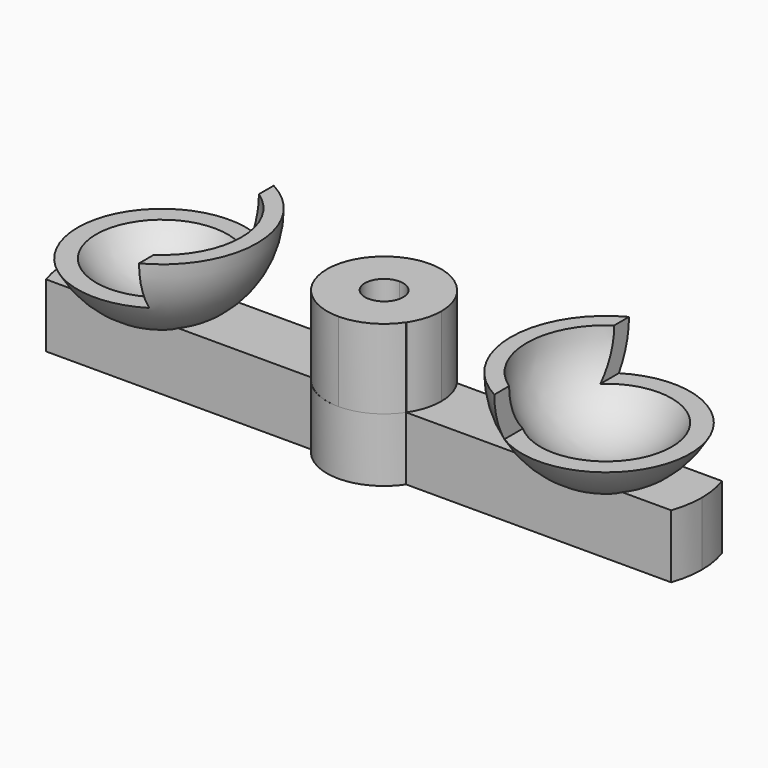
from build123d import *

# Parameters (mm, degrees)
F1_R     = 3
F2_DEPTH = 10
F6_W     = 34.5020639661
F6_H     = 49.154933542
F7_DEPTH = 7
F9_DEPTH = 12.5


with BuildPart() as f2:
    # F1 (on Top) → F2 (new body)
    with BuildSketch(Plane.XY):
        with BuildLine():
            ThreePointArc((46.4564392374, 5), (47.2363289116, 2.5538705461), (47.5, 0))
            ThreePointArc((47.5, 0), (47.2363289116, -2.5538705461), (46.4564392374, -5))
            Line((46.4564392374, -5), (49.2615084811, -5))
            ThreePointArc((49.2615084811, -5), (49.8983064719, -2.5359590739), (50.1125981935, 0))
            ThreePointArc((50.1125981935, 0), (49.8983064719, 2.5359590739), (49.2615084811, 5))
            Line((49.2615084811, 5), (46.4564392374, 5))
        make_face()
        with BuildLine():
            Line((-46.4564392374, 5), (-49.2629836635, 5))
            ThreePointArc((-49.2629836635, 5), (-50.1139903065, 0), (-49.2629836635, -5))
            Line((-49.2629836635, -5), (-46.4564392374, -5))
            ThreePointArc((-46.4564392374, -5), (-47.5, 0), (-46.4564392374, 5))
        make_face()
        with BuildLine():
            ThreePointArc((-22.5, 0), (-22.7636710884, 2.5538705461), (-23.5435607626, 5))
            Line((-23.5435607626, 5), (-46.4564392374, 5))
            ThreePointArc((-46.4564392374, 5), (-47.5, 0), (-46.4564392374, -5))
            Line((-46.4564392374, -5), (-23.5435607626, -5))
            ThreePointArc((-23.5435607626, -5), (-22.7636710884, -2.5538705461), (-22.5, 0))
        make_face()
        with BuildLine():
            ThreePointArc((-19.8860096935, 0), (-20.1002802071, 2.5359521046), (-20.7370163365, 5))
            Line((-20.7370163365, 5), (-23.5435607626, 5))
            ThreePointArc((-23.5435607626, 5), (-22.7636710884, 2.5538705461), (-22.5, 0))
            ThreePointArc((-22.5, 0), (-22.7636710884, -2.5538705461), (-23.5435607626, -5))
            Line((-23.5435607626, -5), (-20.7370163365, -5))
            ThreePointArc((-20.7370163365, -5), (-20.1002802071, -2.5359521046), (-19.8860096935, 0))
        make_face()
        with BuildLine():
            ThreePointArc((-7.4833147735, -5), (-9, 0), (-7.4833147735, 5))
            Line((-7.4833147735, 5), (-20.7370163365, 5))
            ThreePointArc((-20.7370163365, 5), (-20.1002802071, 2.5359521046), (-19.8860096935, 0))
            ThreePointArc((-19.8860096935, 0), (-20.1002802071, -2.5359521046), (-20.7370163365, -5))
            Line((-20.7370163365, -5), (-7.4833147735, -5))
        make_face()
        with BuildLine():
            ThreePointArc((9, 0), (8.6124860802, 2.6124860802), (7.4833147735, 5))
            Line((7.4833147735, 5), (-7.4833147735, 5))
            ThreePointArc((-7.4833147735, 5), (-9, 0), (-7.4833147735, -5))
            Line((-7.4833147735, -5), (7.4833147735, -5))
            ThreePointArc((7.4833147735, -5), (8.6124860802, -2.6124860802), (9, 0))
        make_face()
        Circle(F1_R, mode=Mode.SUBTRACT)
        with BuildLine():
            ThreePointArc((20.7384915189, -5), (19.8874018065, 0), (20.7384915189, 5))
            Line((20.7384915189, 5), (7.4833147735, 5))
            ThreePointArc((7.4833147735, 5), (8.6124860802, 2.6124860802), (9, 0))
            ThreePointArc((9, 0), (8.6124860802, -2.6124860802), (7.4833147735, -5))
            Line((7.4833147735, -5), (20.7384915189, -5))
        make_face()
        with BuildLine():
            ThreePointArc((23.5435607626, -5), (22.5, 0), (23.5435607626, 5))
            Line((23.5435607626, 5), (20.7384915189, 5))
            ThreePointArc((20.7384915189, 5), (19.8874018065, 0), (20.7384915189, -5))
            Line((20.7384915189, -5), (23.5435607626, -5))
        make_face()
        with BuildLine():
            ThreePointArc((46.4564392374, -5), (47.2363289116, -2.5538705461), (47.5, 0))
            ThreePointArc((47.5, 0), (47.2363289116, 2.5538705461), (46.4564392374, 5))
            Line((46.4564392374, 5), (23.5435607626, 5))
            ThreePointArc((23.5435607626, 5), (22.5, 0), (23.5435607626, -5))
            Line((23.5435607626, -5), (46.4564392374, -5))
        make_face()
        with BuildLine():
            Line((-7.4833147735, 5), (7.4833147735, 5))
            ThreePointArc((7.4833147735, 5), (0, 9), (-7.4833147735, 5))
        make_face()
        with BuildLine():
            ThreePointArc((-7.4833147735, -5), (0, -9), (7.4833147735, -5))
            Line((7.4833147735, -5), (-7.4833147735, -5))
        make_face()
    extrude(amount=F2_DEPTH)

    # F8 (on face) → F9 (join)
    with BuildSketch(Plane.XY.offset(10)):
        with BuildLine():
            ThreePointArc((9.0266954303, 0), (8.6391815104, 2.6124860802), (7.5100102038, 5))
            Line((7.5100102038, 5), (7.4833147735, 5))
            ThreePointArc((7.4833147735, 5), (4.2485253114, 7.9341056634), (0.0133477151, 8.9999901021))
            ThreePointArc((0.0133477151, 8.9999901021), (-8.9733045697, 0), (0.0133477151, -8.9999901021))
            ThreePointArc((0.0133477151, -8.9999901021), (4.2485253114, -7.9341056634), (7.4833147735, -5))
            Line((7.4833147735, -5), (7.5100102038, -5))
            ThreePointArc((7.5100102038, -5), (8.6391815104, -2.6124860802), (9.0266954303, 0))
        make_face()
        with BuildLine():
            ThreePointArc((0.0133477151, 2.9999703063), (2.1432913831, 2.126034236), (3.0266954303, 0))
            ThreePointArc((3.0266954303, 0), (2.1432913831, -2.126034236), (0.0133477151, -2.9999703063))
            ThreePointArc((0.0133477151, -2.9999703063), (-3, 0), (0.0133477151, 2.9999703063))
        make_face(mode=Mode.SUBTRACT)
    extrude(amount=F9_DEPTH)


with BuildPart() as f4:
    # F3 (on Front) → F4 (revolve)
    with BuildSketch(Plane.XZ):
        with BuildLine():
            Line((-47.5, 22.5), (-50, 22.5))
            ThreePointArc((-50, 22.5), (-45.6066017178, 11.8933982822), (-35, 7.5))
            Line((-35, 7.5), (-35, 10))
            ThreePointArc((-35, 10), (-43.8388347648, 13.6611652352), (-47.5, 22.5))
        make_face()
    revolve(axis=Axis((-35, 0, 15.5329470341), (0, 0, 1)))


with BuildPart() as f5:
    # F3 (on Front) → F5 (revolve)
    with BuildSketch(Plane.XZ):
        with BuildLine():
            Line((22.5, 22.5), (20, 22.5))
            ThreePointArc((20, 22.5), (24.3933982822, 11.8933982822), (35, 7.5))
            Line((35, 7.5), (35, 10))
            ThreePointArc((35, 10), (26.1611652352, 13.6611652352), (22.5, 22.5))
        make_face()
    revolve(axis=Axis((35, 0, 11.25), (0, 0, -1)))


with BuildPart() as f7_tool:
    # F6 (on face) → F7 (new body)
    with BuildSketch(Plane.XY.offset(22.5)):
        with BuildLine():
            Line((28, 25.6732665002), (28, 13.2664991614))
            ThreePointArc((28, 13.2664991614), (42.7459666924, 12.8452325787), (50, 0))
            ThreePointArc((50, 0), (42.7459666924, -12.8452325787), (28, -13.2664991614))
            Line((28, -13.2664991614), (28, -23.4816670418))
            Line((28, -23.4816670418), (60.3903114407, -23.4816670418))
            Line((60.3903114407, -23.4816670418), (60.3903114407, 25.6732665002))
            Line((60.3903114407, 25.6732665002), (28, 25.6732665002))
        make_face()
        with Locations((-45.251031983, 1.0957997292)):
            Rectangle(F6_W, F6_H)
        with BuildLine():
            Line((28, 10.3561575886), (28, 0))
            Line((28, 0), (28, -10.3561575886))
            ThreePointArc((28, -10.3561575886), (40.8630196998, -11.0397010829), (47.5, 0))
            ThreePointArc((47.5, 0), (40.8630196998, 11.0397010829), (28, 10.3561575886))
        make_face()
        with BuildLine():
            Line((28, 13.2664991614), (28, 10.3561575886))
            ThreePointArc((28, 10.3561575886), (40.8630196998, 11.0397010829), (47.5, 0))
            ThreePointArc((47.5, 0), (40.8630196998, -11.0397010829), (28, -10.3561575886))
            Line((28, -10.3561575886), (28, -13.2664991614))
            ThreePointArc((28, -13.2664991614), (42.7459666924, -12.8452325787), (50, 0))
            ThreePointArc((50, 0), (42.7459666924, 12.8452325787), (28, 13.2664991614))
        make_face()
    extrude(amount=-F7_DEPTH)


with BuildPart() as f4_1:
    add(f4.part)

    # F7: cut by f7_tool
    add(f7_tool.part, mode=Mode.SUBTRACT)


with BuildPart() as f5_1:
    add(f5.part)

    # F7: cut by f7_tool
    add(f7_tool.part, mode=Mode.SUBTRACT)


solid = Compound([f2.part, f4_1.part, f5_1.part])
